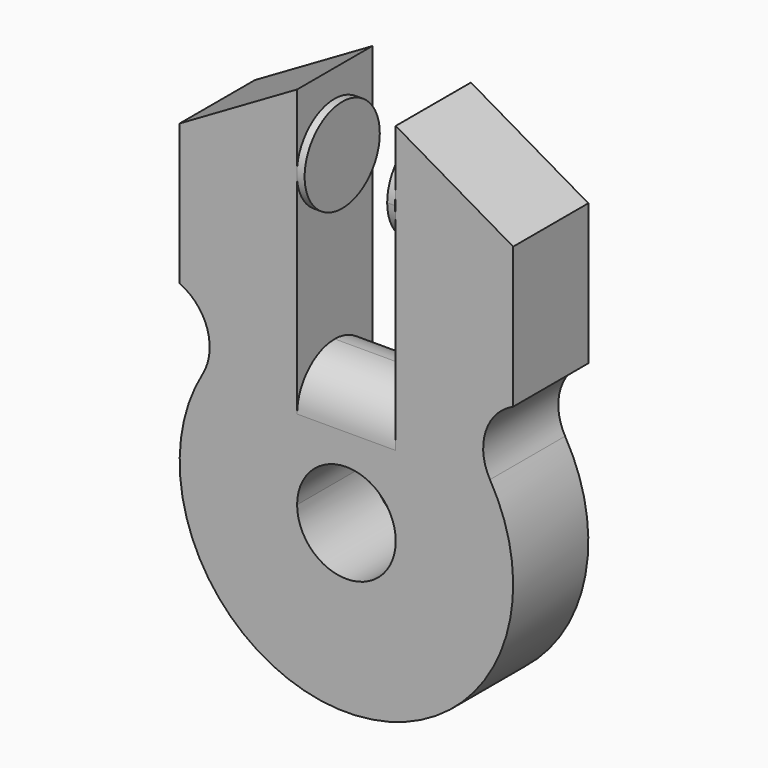
from build123d import *

# Parameters (mm, degrees)
F1_DEPTH = 6
F3_DEPTH = 0.5
F4_R     = 3
F5_DEPTH = 0.5
F6_DEPTH = 6
F7_R     = 3
F8_R     = 2.99999


# Not quite as in the source:
# - a fillet or chamfer is up to 0.001 mm smaller than in the source, because OpenCascade refuses the exact size


with BuildPart() as f1:
    # F0 (on Front) → F1 (new body)
    with BuildSketch(Plane.XZ):
        with BuildLine():
            Line((-38.9118868113, 40.6996482372), (-38.9118868113, 42.7731432119))
            ThreePointArc((-38.9118868113, 42.7731432119), (-42.3638979782, 40.9564388024), (-44.9301813825, 38.0185849093))
            ThreePointArc((-44.9301813825, 38.0185849093), (-35.7618868113, 21.9496482372), (-26.59359224, 38.0185849093))
            ThreePointArc((-26.59359224, 38.0185849093), (-29.1598756443, 40.9564388024), (-32.6118868113, 42.7731432119))
            Line((-32.6118868113, 42.7731432119), (-32.6118868113, 40.6996482372))
            Line((-32.6118868113, 40.6996482372), (-35.7618868113, 40.6996482372))
            Line((-35.7618868113, 40.6996482372), (-38.9118868113, 40.6996482372))
        make_face()
        with BuildLine():
            ThreePointArc((-35.7618868113, 35.7496482372), (-33.5345004505, 34.827034598), (-32.6118868113, 32.5996482372))
            ThreePointArc((-32.6118868113, 32.5996482372), (-35.7618868113, 29.4496482372), (-38.9118868113, 32.5996482372))
            ThreePointArc((-38.9118868113, 32.5996482372), (-37.989273172, 34.827034598), (-35.7618868113, 35.7496482372))
        make_face(mode=Mode.SUBTRACT)
        with BuildLine():
            ThreePointArc((-44.9301813825, 38.0185849093), (-42.3638979782, 40.9564388024), (-38.9118868113, 42.7731432119))
            Line((-38.9118868113, 42.7731432119), (-38.9118868113, 55.9496482372))
            Line((-38.9118868113, 55.9496482372), (-46.4118868113, 51.5996482372))
            Line((-46.4118868113, 51.5996482372), (-46.4118868113, 42.5996482372))
            ThreePointArc((-46.4118868113, 42.5996482372), (-44.652769306, 40.6384655389), (-44.9301813825, 38.0185849093))
        make_face()
        with BuildLine():
            ThreePointArc((-32.6118868113, 42.7731432119), (-29.1598756443, 40.9564388024), (-26.59359224, 38.0185849093))
            ThreePointArc((-26.59359224, 38.0185849093), (-26.8710043165, 40.6384655389), (-25.1118868113, 42.5996482372))
            Line((-25.1118868113, 42.5996482372), (-25.1118868113, 51.5996482372))
            Line((-25.1118868113, 51.5996482372), (-32.6118868113, 55.9496482372))
            Line((-32.6118868113, 55.9496482372), (-32.6118868113, 42.7731432119))
        make_face()
    extrude(amount=F1_DEPTH)

    # F2 (on face) → F3 (join)
    with BuildSketch(Plane(origin=(-32.6118868113, 0, 0), x_dir=(0, -1, 0), z_dir=(-1, 0, 0))):
        with BuildLine():
            ThreePointArc((3, 54.4897693761), (0.9582631067, 49.3483636635), (6.0587201472, 51.4903441072))
            ThreePointArc((6.0587201472, 51.4903441072), (5.1591771878, 53.6323245508), (3, 54.4897693761))
        make_face()
    extrude(amount=F3_DEPTH)

    # F4 (on face) → F5 (join)
    with BuildSketch(Plane.YZ.offset(-38.9118868113)):
        with Locations((-3.0229054391, 51.2129813433)):
            Circle(F4_R)
    extrude(amount=F5_DEPTH)

    # F0 (on Front) → F6 (join)
    with BuildSketch(Plane.XZ):
        with BuildLine():
            Line((-38.9118868113, 40.6996482372), (-38.9118868113, 42.7731432119))
            ThreePointArc((-38.9118868113, 42.7731432119), (-42.3638979782, 40.9564388024), (-44.9301813825, 38.0185849093))
            ThreePointArc((-44.9301813825, 38.0185849093), (-35.7618868113, 21.9496482372), (-26.59359224, 38.0185849093))
            ThreePointArc((-26.59359224, 38.0185849093), (-29.1598756443, 40.9564388024), (-32.6118868113, 42.7731432119))
            Line((-32.6118868113, 42.7731432119), (-32.6118868113, 40.6996482372))
            Line((-32.6118868113, 40.6996482372), (-35.7618868113, 40.6996482372))
            Line((-35.7618868113, 40.6996482372), (-38.9118868113, 40.6996482372))
        make_face()
        with BuildLine():
            ThreePointArc((-35.7618868113, 35.7496482372), (-33.5345004505, 34.827034598), (-32.6118868113, 32.5996482372))
            ThreePointArc((-32.6118868113, 32.5996482372), (-35.7618868113, 29.4496482372), (-38.9118868113, 32.5996482372))
            ThreePointArc((-38.9118868113, 32.5996482372), (-37.989273172, 34.827034598), (-35.7618868113, 35.7496482372))
        make_face(mode=Mode.SUBTRACT)
        with BuildLine():
            ThreePointArc((-44.9301813825, 38.0185849093), (-42.3638979782, 40.9564388024), (-38.9118868113, 42.7731432119))
            Line((-38.9118868113, 42.7731432119), (-38.9118868113, 55.9496482372))
            Line((-38.9118868113, 55.9496482372), (-46.4118868113, 51.5996482372))
            Line((-46.4118868113, 51.5996482372), (-46.4118868113, 42.5996482372))
            ThreePointArc((-46.4118868113, 42.5996482372), (-44.652769306, 40.6384655389), (-44.9301813825, 38.0185849093))
        make_face()
        with BuildLine():
            ThreePointArc((-32.6118868113, 42.7731432119), (-29.1598756443, 40.9564388024), (-26.59359224, 38.0185849093))
            ThreePointArc((-26.59359224, 38.0185849093), (-26.8710043165, 40.6384655389), (-25.1118868113, 42.5996482372))
            Line((-25.1118868113, 42.5996482372), (-25.1118868113, 51.5996482372))
            Line((-25.1118868113, 51.5996482372), (-32.6118868113, 55.9496482372))
            Line((-32.6118868113, 55.9496482372), (-32.6118868113, 42.7731432119))
        make_face()
    extrude(amount=F6_DEPTH)

    # F7
    f7_edges = [f1.edges().sort_by_distance(p)[0] for p in [
        (-35.761887, -6, 40.699648),
    ]]
    fillet(f7_edges, radius=F7_R)

    # F8 (radius 3 in the source; OpenCascade refuses exactly that, so slightly less here)
    f8_edges = [f1.edges().sort_by_distance(p)[0] for p in [
        (-35.761887, 0, 40.699648),
    ]]
    fillet(f8_edges, radius=F8_R)


solid = f1.part
